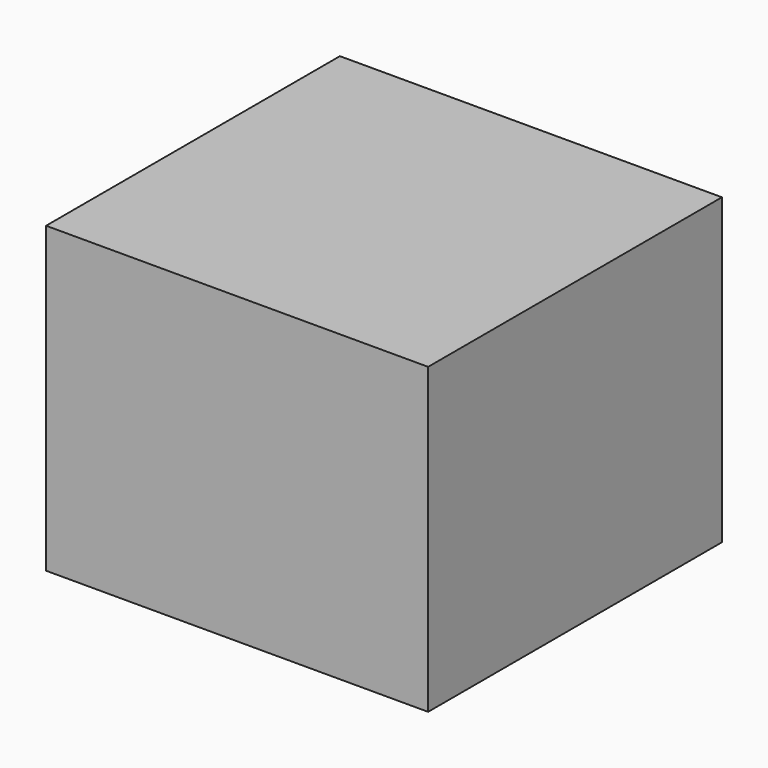
from build123d import *

# Parameters (mm, degrees)
F0_W      = 63.8971067965
F0_H      = 61.4244844764
F1_DEPTH  = 25.4
F2_R      = 20.9044969904
F1_FACE_W = 63.8971067965
F1_FACE_H = 61.4244844764
F3_DEPTH  = 25.4


# Not quite as in the source:
# - a feature of the source that left no trace in its solid (it failed there, or was rolled back) is left out


with BuildPart() as f1:
    # F0 (on Top) → F1 (new body)
    with BuildSketch(Plane.XY):
        with Locations((-7.7395718545, 2.0738141611)):
            Rectangle(F0_W, F0_H)
    extrude(amount=F1_DEPTH)

    # F2 (on Top) + F1_face (on face) → F3 (join)
    with BuildSketch(Plane.XY):
        with Locations((-32.6551906765, 39.2090491951)):
            Circle(F2_R)
    with BuildSketch(Plane(origin=(-7.7395718545, 2.0738141611, 25.4), x_dir=(1, 0, 0), z_dir=(0, 0, 1))):
        Rectangle(F1_FACE_W, F1_FACE_H)
    extrude(amount=F3_DEPTH)


solid = f1.part
